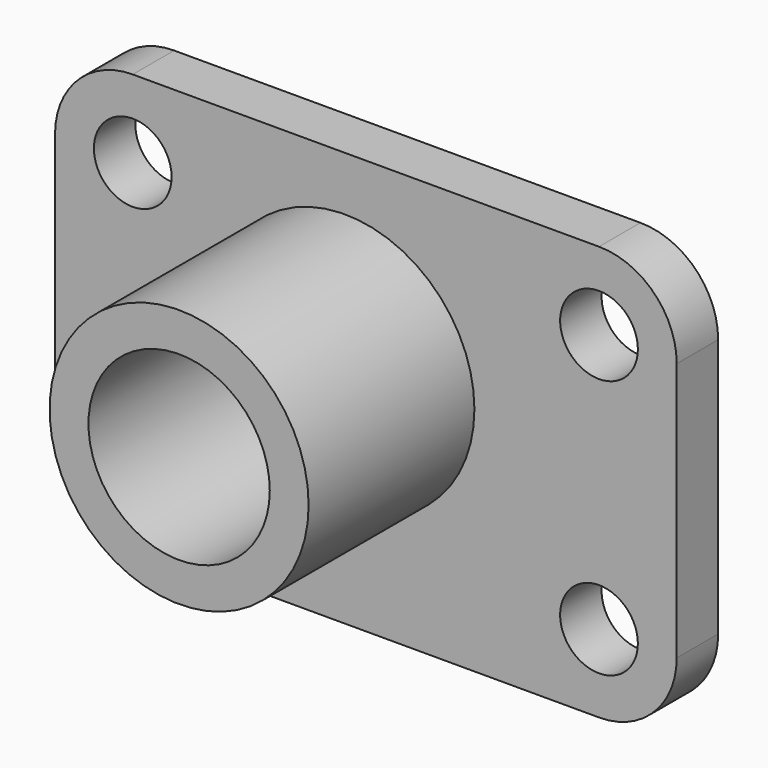
from build123d import *

# Parameters (mm, degrees)
F0_R     = 25
F0_R_2   = 17.5
F1_DEPTH = 50
F2_DEPTH = 112
F0_R_3   = 7.5
F3_DEPTH = 10


# Not quite as in the source:
# - an extrude ends at something that could not be found from the text; its depth is read off the source's solid


with BuildPart() as f1:
    # F0 (on Front) → F1 (new body)
    with BuildSketch(Plane.XZ):
        Circle(F0_R)
        Circle(F0_R_2, mode=Mode.SUBTRACT)
    extrude(amount=F1_DEPTH)

    # F0 (on Front) → F2 (cut, through all)
    with BuildSketch(Plane.XZ):
        Circle(F0_R_2)
    extrude(amount=-F2_DEPTH, mode=Mode.SUBTRACT)

    # F0 (on Front) → F3 (join)
    with BuildSketch(Plane.XZ):
        with BuildLine():
            Line((49.0495060384, 35.4441977432), (-40.9504939616, 35.4441977432))
            ThreePointArc((-40.9504939616, 35.4441977432), (-51.5570956794, 31.050799461), (-55.9504939616, 20.4441977432))
            Line((-55.9504939616, 20.4441977432), (-55.9504939616, -29.5558022568))
            ThreePointArc((-55.9504939616, -29.5558022568), (-51.5570956794, -40.1624039746), (-40.9504939616, -44.5558022568))
            Line((-40.9504939616, -44.5558022568), (49.0495060384, -44.5558022568))
            ThreePointArc((49.0495060384, -44.5558022568), (59.6561077562, -40.1624039746), (64.0495060384, -29.5558022568))
            Line((64.0495060384, -29.5558022568), (64.0495060384, 20.4441977432))
            ThreePointArc((64.0495060384, 20.4441977432), (59.6561077562, 31.050799461), (49.0495060384, 35.4441977432))
        make_face()
        with Locations((-40.9504939616, -29.5558022568)):
            Circle(F0_R_3, mode=Mode.SUBTRACT)
        with Locations((49.0495060384, -29.5558022568)):
            Circle(F0_R_3, mode=Mode.SUBTRACT)
        Circle(F0_R, mode=Mode.SUBTRACT)
        with Locations((-40.9504939616, 20.4441977432)):
            Circle(F0_R_3, mode=Mode.SUBTRACT)
        with Locations((49.0495060384, 20.4441977432)):
            Circle(F0_R_3, mode=Mode.SUBTRACT)
    extrude(amount=F3_DEPTH)


solid = f1.part
